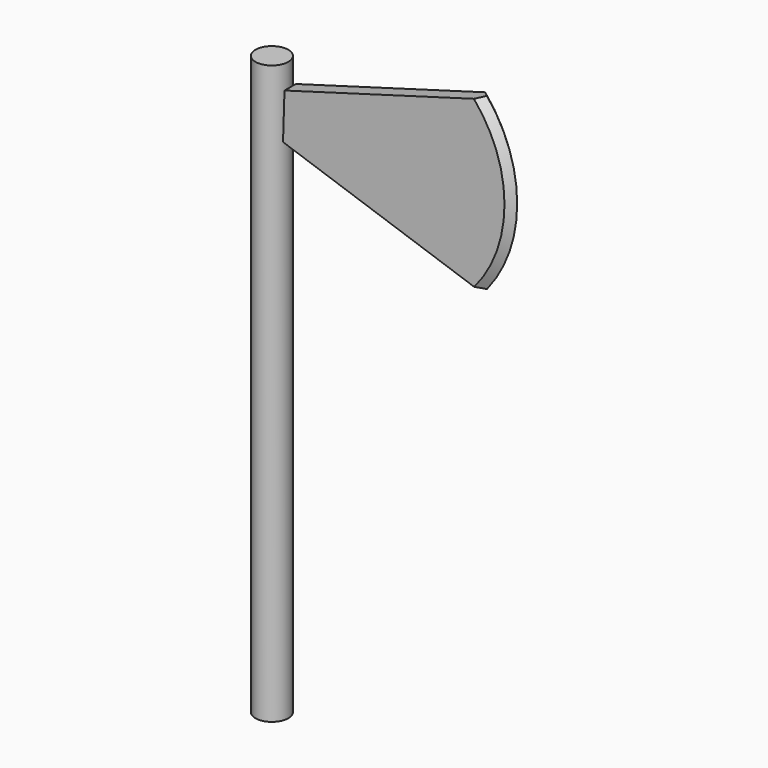
from build123d import *

# Parameters (mm, degrees)
F0_R          = 9.525
F1_DEPTH      = 334.85178
F3_DEPTH      = 4.18014
F3_DEPTH_BACK = 3.99072
F4_T2_ANGLE   = 96.5800048024
F4_T4_ANGLE   = 96.5800048024


# Not quite as in the source:
# - a fillet or chamfer that OpenCascade refuses, or shapes differently, is made with other operations: its cross-section is extruded or revolved along the edge and cut away or added


with BuildPart() as f1:
    # F0 (on Top) → F1 (new body)
    with BuildSketch(Plane.XY):
        Circle(F0_R)
    extrude(amount=F1_DEPTH)


with BuildPart() as f3:
    # F2 (on Front) → F3 (new body, two sides)
    with BuildSketch(Plane.XZ) as f3_sk:
        with BuildLine():
            Line((125.7524490356, 355.3073406219), (10.6634572148, 322.3180174828))
            Line((10.6634572148, 322.3180174828), (9.8127294332, 295.7464158535))
            Line((9.8127294332, 295.7464158535), (125.7524490356, 256.1295628548))
            ThreePointArc((125.7524490356, 256.1295628548), (143.2271122484, 305.7184517384), (125.7524490356, 355.3073406219))
        make_face()
    extrude(amount=F3_DEPTH)
    extrude(f3_sk.sketch, amount=-F3_DEPTH_BACK)

    # F4: chamfer of 5.08 on 2 edges, made by hand

    # F4_s1 → F4_t2 (revolve, cut)
    with BuildSketch(Plane(origin=(187.5911639165, 0, 167.1963566243), x_dir=(0, 1, 0), z_dir=(-0.7465220942, 0, -0.6653606262))):
        Polygon((0.89986, -106.4585931816), (-4.18014, -111.5385931816), (-4.18014, -106.4585931816), align=None)
    revolve(axis=Axis((64.129114151, -4.18014, 305.7184517384), (0, -1, 0)), revolution_arc=F4_T2_ANGLE, mode=Mode.SUBTRACT)

    # F4_s3 → F4_t4 (revolve, cut)
    with BuildSketch(Plane(origin=(187.5911639165, 0, 167.1963566243), x_dir=(0, 1, 0), z_dir=(-0.7465220942, 0, -0.6653606262))):
        Polygon((-1.08928, -106.4585931816), (3.99072, -111.5385931816), (3.99072, -106.4585931816), align=None)
    revolve(axis=Axis((64.129114151, 3.99072, 305.7184517384), (0, -1, 0)), revolution_arc=F4_T4_ANGLE, mode=Mode.SUBTRACT)


solid = Compound([f1.part, f3.part])
